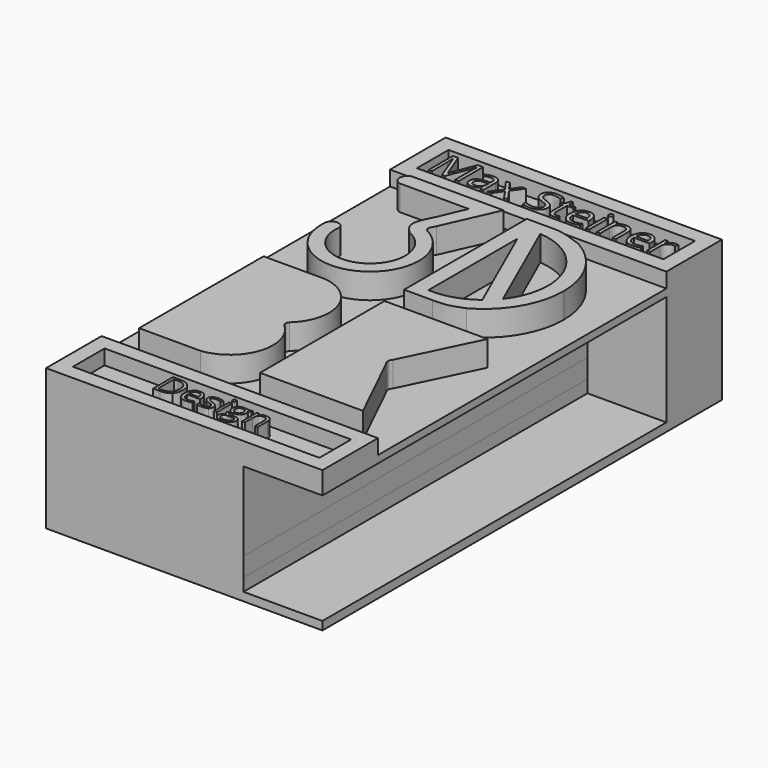
from build123d import *

# Parameters (mm, degrees)
F1_W         = 55.6107703596
F1_H         = 92.8997322917
F2_DEPTH     = 25.4
F3_DEPTH     = 5.08
F4_TEXT_SIZE = 8.577041121
F5_DEPTH     = 3
F4_W         = 0.5673257474
F4_H         = 3.7439126875
F6_DEPTH     = 3
F7_W         = 55.6107703596
F7_H         = 3.7946861994
F8_DEPTH     = 25.4
F9_W         = 55.6107703596
F9_H         = 3.7949544203
F10_DEPTH    = 25.4
F11_W        = 15.875
F11_H        = 7.9375
F11_W_2      = 15.8749995753
F11_H_2      = 3.81
F12_DEPTH    = 86.5193729115


# Not quite as in the source:
# - ends of sketch curves that miss each other by under 0.0002 mm in the source are joined
# - Text() gives the source's letters only with a copy of the font that has no kerning and outlines rounded to 1/6400 em; it was checked with that copy


with BuildPart() as f2:
    # F1 (on Top) → F2 (new body)
    with BuildSketch(Plane.XY):
        with Locations((-0.0001015142, 0.0001341105)):
            Rectangle(F1_W, F1_H)
    extrude(amount=-F2_DEPTH)

    # F0 (on Top) → F3 (join)
    with BuildSketch(Plane.XY):
        with BuildLine():
            Line((1.9535701722, 33.4806852043), (1.9535701722, 2.6171170175))
            Line((1.9535701722, 2.6171170175), (7.6673883013, 2.6171170175))
            add(Edge.make_bspline(
                [(13.5640528841, 3.8033656441), (12.5585792201, 3.4051600509), (10.5947152477, 2.6273956539), (8.6274422547, 2.6204880265), (7.6673883013, 2.6171170175)],
                knots=[0, 0, 0, 0, 0.5119874279, 1, 1, 1, 1], degree=3))
            ThreePointArc((13.5640528841, 3.8033656441), (19.5771167094, 9.6257290209), (21.8482203782, 17.6817168551))
            Line((21.8482203782, 17.6817168551), (21.8482203782, 18.0489011109))
            ThreePointArc((21.8482203782, 18.0489011109), (19.5771167094, 26.1048889451), (13.5640528841, 31.9272523219))
            add(Edge.make_bspline(
                [(13.5640528841, 31.9272523219), (12.0188625137, 32.4806988664), (9.5071250594, 33.3803371514), (8.1786150797, 33.4528004476), (7.6673883013, 33.4806852043)],
                knots=[0, 0, 0, 0, 0.6151878524, 1, 1, 1, 1], degree=3))
            Line((7.6673883013, 33.4806852043), (1.9535701722, 33.4806852043))
        make_face()
        with BuildLine():
            ThreePointArc((13.7255926495, 7.5781230036), (9.6198125415, 5.4448354943), (5.0269701927, 4.8843490524))
            Line((5.0269701927, 4.8843490524), (5.0269701927, 27.2558980547))
            Line((5.0269701927, 27.2558980547), (13.7255926495, 7.5781230036))
        make_face(mode=Mode.SUBTRACT)
        with BuildLine():
            ThreePointArc((6.7811124511, 30.8286115181), (17.6657420253, 23.1223286699), (16.0391214303, 9.8854082672))
            Line((16.0391214303, 9.8854082672), (6.7811124511, 30.8286115181))
        make_face(mode=Mode.SUBTRACT)
        with BuildLine():
            Line((-7.5453622267, 22.6989928633), (-2.7351737954, 33.4806852043))
            Line((-2.7351737954, 33.4806852043), (-21.1572051048, 33.4806852043))
            ThreePointArc((-21.1572051048, 33.4806852043), (-22.3890896886, 31.9530339911), (-21.1572051048, 30.425382778))
            Line((-21.1572051048, 30.425382778), (-7.2931135073, 30.425382778))
            Line((-7.2931135073, 30.425382778), (-9.4495294616, 25.3879800439))
            add(Edge.make_bspline(
                [(-9.4495294616, 25.3879800439), (-10.3302159731, 23.6726618568), (-11.8808970013, 20.6523914937), (-10.1830913379, 19.0052173822), (-9.4495294616, 18.2935316116)],
                knots=[0, 0, 0, 0, 0.5679353107, 1, 1, 1, 1], degree=3))
            ThreePointArc((-9.4495294616, 18.2935316116), (-8.744805336, 5.5966861339), (-19.1914085299, 12.8475483507))
            ThreePointArc((-19.1914085299, 12.8475483507), (-20.5873309935, 13.9352987723), (-21.9832534571, 12.8475483507))
            ThreePointArc((-21.9832534571, 12.8475483507), (-7.5716745464, 3.0830422585), (-7.6246123494, 20.4909825018))
            add(Edge.make_bspline(
                [(-7.5453622267, 22.6989928633), (-7.8757345138, 22.1285959519), (-8.4306078493, 21.1705917574), (-7.8693930702, 20.681447967), (-7.6246123494, 20.4909825018)],
                knots=[0, 0, 0, 0, 0.5706142153, 0.9583691649, 0.9583691649, 0.9583691649, 0.9583691649], degree=3))
        make_face()
        with BuildLine():
            Line((1.9535701722, -33.6182080209), (21.8482203782, -33.6182080209))
            Line((21.8482203782, -33.6182080209), (22.670282051, -33.6182080209))
            Line((22.670282051, -33.6182080209), (15.4876355082, -18.8196848612))
            add(Edge.make_bspline(
                [(15.4876355082, -18.8196848612), (15.371168109, -18.6560732739), (15.159509665, -18.3587387901), (15.1679139181, -18.0863425739), (15.171693638, -17.9638353875)],
                knots=[0, 0, 0, 0, 0.550261057, 1, 1, 1, 1], degree=3))
            add(Edge.make_bspline(
                [(15.4876355082, -17.1079859138), (15.371168109, -17.2715975011), (15.159509665, -17.5689319849), (15.1679139181, -17.8413282011), (15.171693638, -17.9638353875)],
                knots=[0, 0, 0, 0, 0.550261057, 1, 1, 1, 1], degree=3))
            Line((15.4876355082, -17.1079859138), (22.670282051, -2.3094627541))
            Line((22.670282051, -2.3094627541), (1.9535701722, -2.3094627541))
            Line((1.9535701722, -2.3094627541), (1.9535701722, -33.6182080209))
        make_face()
        with BuildLine():
            Line((-22.3890896886, -2.3094627541), (-22.3890896886, -33.6182080209))
            Line((-22.3890896886, -33.6182080209), (-10.0687015802, -33.6182080209))
            ThreePointArc((-10.0687015802, -33.6182080209), (-2.7489802993, -27.706179837), (-5.1699676551, -18.6139184516))
            add(Edge.make_bspline(
                [(-5.1699676551, -18.6139184516), (-5.2577137292, -18.4897791328), (-5.4173213156, -18.2639732804), (-5.4122223799, -18.0570156997), (-5.4099266417, -17.9638353875)],
                knots=[0, 0, 0, 0, 0.5497612996, 1, 1, 1, 1], degree=3))
            add(Edge.make_bspline(
                [(-5.1699676551, -17.3137523234), (-5.2577137292, -17.4378916422), (-5.4173213156, -17.6636974946), (-5.4122223799, -17.8706550753), (-5.4099266417, -17.9638353875)],
                knots=[0, 0, 0, 0, 0.5497612996, 1, 1, 1, 1], degree=3))
            ThreePointArc((-5.1699676551, -17.3137523234), (-2.7489802993, -8.221490938), (-10.0687015802, -2.3094627541))
            Line((-10.0687015802, -2.3094627541), (-22.3890896886, -2.3094627541))
        make_face()
    extrude(amount=F3_DEPTH)

    # F4 (on face) → F5 (join)
    with BuildSketch(Plane.XY):
        with Locations((-23.8402802497, 39.9415232241)):
            Text('Max Steiner', F4_TEXT_SIZE, font='Open Sans', text_align=(TextAlign.LEFT, TextAlign.BOTTOM))
        Polygon((-27.805486694, 46.4500002563), (-27.805486694, 36.2746864557), (27.8052836657, 36.2746864557), (27.8052836657, 46.4500002563), (24.8052836657, 46.4500002563), (24.8052836657, 39.2746864557), (-24.805486694, 39.2746864557), (-24.805486694, 46.4500002563), align=None)
        Polygon((-27.805486694, 50.2446864557), (-27.805486694, 46.4500002563), (-24.805486694, 46.4500002563), (-24.805486694, 47.2446864557), (24.8052836657, 47.2446864557), (24.8052836657, 46.4500002563), (27.8052836657, 46.4500002563), (27.8052836657, 50.2446864557), align=None)
    extrude(amount=F5_DEPTH)

    # F4 (on face) → F6 (join)
    with BuildSketch(Plane.XY):
        Polygon((27.8052836657, -36.2746864557), (-27.805486694, -36.2746864557), (-27.805486694, -46.4497320354), (-24.805486694, -46.4497320354), (-24.805486694, -39.2746864557), (24.8052836657, -39.2746864557), (24.8052836657, -46.4497320354), (27.8052836657, -46.4497320354), align=None)
        Polygon((-24.805486694, -46.4497320354), (-27.805486694, -46.4497320354), (-27.805486694, -50.2446864557), (27.8052836657, -50.2446864557), (27.8052836657, -46.4497320354), (24.8052836657, -46.4497320354), (24.8052836657, -47.2446864557), (-24.805486694, -47.2446864557), align=None)
        with BuildLine():
            add(Edge.make_bspline(
                [(-6.3295820825, -42.6227643038), (-6.3295820825, -43.8590753256), (-7.0007535833, -44.5133035719)],
                knots=[0, 0, 0, 1, 1, 1], degree=2))
            add(Edge.make_bspline(
                [(-6.9750654232, -40.818580978), (-6.3295820825, -41.4640643188), (-6.3295820825, -42.6227643038)],
                knots=[0, 0, 0, 1, 1, 1], degree=2))
            add(Edge.make_bspline(
                [(-8.7858074282, -40.1730976373), (-7.620548764, -40.1730976373), (-6.9750654232, -40.818580978)],
                knots=[0, 0, 0, 1, 1, 1], degree=2))
            Line((-8.7858074282, -40.1730976373), (-10.316165899, -40.1730976373))
            Line((-10.316165899, -40.1730976373), (-10.316165899, -45.1675318182))
            Line((-10.316165899, -45.1675318182), (-8.9322845961, -45.1675318182))
            add(Edge.make_bspline(
                [(-7.0007535833, -44.5133035719), (-7.671925084, -45.1675318182), (-8.9322845961, -45.1675318182)],
                knots=[0, 0, 0, 1, 1, 1], degree=2))
        make_face()
        with BuildLine():
            add(Edge.make_bspline(
                [(-6.9439116972, -42.6435334545), (-6.9439116972, -41.6662902596), (-7.4341729645, -41.1711099829)],
                knots=[0, 0, 0, 1, 1, 1], degree=2))
            add(Edge.make_bspline(
                [(-7.4669663603, -44.1547624444), (-6.9439116972, -43.6437320265), (-6.9439116972, -42.6435334545)],
                knots=[0, 0, 0, 1, 1, 1], degree=2))
            add(Edge.make_bspline(
                [(-9.0284785571, -44.6657928624), (-7.9900210233, -44.6657928624), (-7.4669663603, -44.1547624444)],
                knots=[0, 0, 0, 1, 1, 1], degree=2))
            Line((-9.0284785571, -44.6657928624), (-9.7357227933, -44.6657928624))
            Line((-9.7357227933, -44.6657928624), (-9.7357227933, -40.6759297063))
            Line((-9.7357227933, -40.6759297063), (-8.8918394079, -40.6759297063))
            add(Edge.make_bspline(
                [(-7.4341729645, -41.1711099829), (-7.9244342317, -40.6759297063), (-8.8918394079, -40.6759297063)],
                knots=[0, 0, 0, 1, 1, 1], degree=2))
        make_face(mode=Mode.SUBTRACT)
        with BuildLine():
            add(Edge.make_bspline(
                [(-3.7192277766, -45.2363979493), (-4.5489006904, -45.2363979493), (-5.0293239389, -44.7302865408)],
                knots=[0, 0, 0, 1, 1, 1], degree=2))
            add(Edge.make_bspline(
                [(-3.072104766, -45.1795560633), (-3.3399174984, -45.2363979493), (-3.7192277766, -45.2363979493)],
                knots=[0, 0, 0, 1, 1, 1], degree=2))
            add(Edge.make_bspline(
                [(-2.5036859054, -44.9937268204), (-2.8042920336, -45.1227141772), (-3.072104766, -45.1795560633)],
                knots=[0, 0, 0, 1, 1, 1], degree=2))
            Line((-2.5036859054, -44.9937268204), (-2.5036859054, -44.4876154118))
            add(Edge.make_bspline(
                [(-3.6984586259, -44.7401245595), (-3.0939670299, -44.7401245595), (-2.5036859054, -44.4876154118)],
                knots=[0, 0, 0, 1, 1, 1], degree=2))
            add(Edge.make_bspline(
                [(-4.5882527653, -44.3985266866), (-4.2723430524, -44.7401245595), (-3.6984586259, -44.7401245595)],
                knots=[0, 0, 0, 1, 1, 1], degree=2))
            add(Edge.make_bspline(
                [(-4.9216522893, -43.397781558), (-4.9041624782, -44.0569288136), (-4.5882527653, -44.3985266866)],
                knots=[0, 0, 0, 1, 1, 1], degree=2))
            Line((-4.9216522893, -43.397781558), (-2.342998266, -43.397781558))
            Line((-2.342998266, -43.397781558), (-2.342998266, -43.0392404305))
            add(Edge.make_bspline(
                [(-2.7529157135, -41.8176864368), (-2.342998266, -42.2806198743), (-2.342998266, -43.0392404305)],
                knots=[0, 0, 0, 1, 1, 1], degree=2))
            add(Edge.make_bspline(
                [(-3.8657049445, -41.3547529994), (-3.1628331611, -41.3547529994), (-2.7529157135, -41.8176864368)],
                knots=[0, 0, 0, 1, 1, 1], degree=2))
            add(Edge.make_bspline(
                [(-5.0637570045, -41.8876456812), (-4.6177668216, -41.3547529994), (-3.8657049445, -41.3547529994)],
                knots=[0, 0, 0, 1, 1, 1], degree=2))
            add(Edge.make_bspline(
                [(-5.5097471874, -43.3267292004), (-5.5097471874, -42.420538363), (-5.0637570045, -41.8876456812)],
                knots=[0, 0, 0, 1, 1, 1], degree=2))
            add(Edge.make_bspline(
                [(-5.0293239389, -44.7302865408), (-5.5097471874, -44.2241751322), (-5.5097471874, -43.3267292004)],
                knots=[0, 0, 0, 1, 1, 1], degree=2))
        make_face()
        with BuildLine():
            add(Edge.make_bspline(
                [(-3.8733567368, -41.8302572386), (-4.3237193725, -41.8302572386), (-4.5920786615, -42.123758131)],
                knots=[0, 0, 0, 1, 1, 1], degree=2))
            add(Edge.make_bspline(
                [(-3.1896144343, -42.1155597821), (-3.4284596671, -41.8302572386), (-3.8733567368, -41.8302572386)],
                knots=[0, 0, 0, 1, 1, 1], degree=2))
            add(Edge.make_bspline(
                [(-2.9507692016, -42.9364877903), (-2.9507692016, -42.4008623255), (-3.1896144343, -42.1155597821)],
                knots=[0, 0, 0, 1, 1, 1], degree=2))
            Line((-2.9507692016, -42.9364877903), (-4.908534931, -42.9364877903))
            add(Edge.make_bspline(
                [(-4.5920786615, -42.123758131), (-4.8604379505, -42.4172590234), (-4.908534931, -42.9364877903)],
                knots=[0, 0, 0, 1, 1, 1], degree=2))
        make_face(mode=Mode.SUBTRACT)
        with BuildLine():
            add(Edge.make_bspline(
                [(1.0390939545, -44.1465640955), (1.0390939545, -44.6690722019), (0.6499456576, -44.9527350756)],
                knots=[0, 0, 0, 1, 1, 1], degree=2))
            add(Edge.make_bspline(
                [(0.8051677311, -43.527862028), (1.0390939545, -43.7738124965), (1.0390939545, -44.1465640955)],
                knots=[0, 0, 0, 1, 1, 1], degree=2))
            add(Edge.make_bspline(
                [(-0.0944644271, -43.0392404305), (0.5712415077, -43.2819115595), (0.8051677311, -43.527862028)],
                knots=[0, 0, 0, 1, 1, 1], degree=2))
            add(Edge.make_bspline(
                [(-0.7503323432, -42.762136236), (-0.579806685, -42.8577836404), (-0.0944644271, -43.0392404305)],
                knots=[0, 0, 0, 1, 1, 1], degree=2))
            add(Edge.make_bspline(
                [(-0.9979224815, -42.5610034084), (-0.9208580013, -42.6664888316), (-0.7503323432, -42.762136236)],
                knots=[0, 0, 0, 1, 1, 1], degree=2))
            add(Edge.make_bspline(
                [(-1.0749869616, -42.3046683645), (-1.0749869616, -42.4555179852), (-0.9979224815, -42.5610034084)],
                knots=[0, 0, 0, 1, 1, 1], degree=2))
            add(Edge.make_bspline(
                [(-0.8700282378, -41.9565118124), (-1.0749869616, -42.0827663863), (-1.0749869616, -42.3046683645)],
                knots=[0, 0, 0, 1, 1, 1], degree=2))
            add(Edge.make_bspline(
                [(-0.2617107457, -41.8302572386), (-0.6650695141, -41.8302572386), (-0.8700282378, -41.9565118124)],
                knots=[0, 0, 0, 1, 1, 1], degree=2))
            add(Edge.make_bspline(
                [(0.759256977, -42.0619972356), (0.1963036824, -41.8302572386), (-0.2617107457, -41.8302572386)],
                knots=[0, 0, 0, 1, 1, 1], degree=2))
            Line((0.759256977, -42.0619972356), (0.9614829178, -41.6007034679))
            add(Edge.make_bspline(
                [(-0.2212655575, -41.3547529994), (0.3832260384, -41.3547529994), (0.9614829178, -41.6007034679)],
                knots=[0, 0, 0, 1, 1, 1], degree=2))
            add(Edge.make_bspline(
                [(-1.2422332802, -41.6198329488), (-0.8694816812, -41.3547529994), (-0.2212655575, -41.3547529994)],
                knots=[0, 0, 0, 1, 1, 1], degree=2))
            add(Edge.make_bspline(
                [(-1.6149848792, -42.3429273263), (-1.6149848792, -41.8849128982), (-1.2422332802, -41.6198329488)],
                knots=[0, 0, 0, 1, 1, 1], degree=2))
            add(Edge.make_bspline(
                [(-1.5073132296, -42.7829053867), (-1.6149848792, -42.5987158136), (-1.6149848792, -42.3429273263)],
                knots=[0, 0, 0, 1, 1, 1], degree=2))
            add(Edge.make_bspline(
                [(-1.1793792716, -43.1124790145), (-1.3996415801, -42.9670949597), (-1.5073132296, -42.7829053867)],
                knots=[0, 0, 0, 1, 1, 1], degree=2))
            add(Edge.make_bspline(
                [(-0.4366088566, -43.4524372176), (-0.9591169631, -43.2578630692), (-1.1793792716, -43.1124790145)],
                knots=[0, 0, 0, 1, 1, 1], degree=2))
            add(Edge.make_bspline(
                [(0.3034287753, -43.8197232506), (0.1143201929, -43.6645011772), (-0.4366088566, -43.4524372176)],
                knots=[0, 0, 0, 1, 1, 1], degree=2))
            add(Edge.make_bspline(
                [(0.4925373578, -44.1935679628), (0.4925373578, -43.9749453241), (0.3034287753, -43.8197232506)],
                knots=[0, 0, 0, 1, 1, 1], degree=2))
            add(Edge.make_bspline(
                [(0.253692125, -44.6258942308), (0.4925373578, -44.4843360722), (0.4925373578, -44.1935679628)],
                knots=[0, 0, 0, 1, 1, 1], degree=2))
            add(Edge.make_bspline(
                [(-0.4289570643, -44.7674523894), (0.0148468923, -44.7674523894), (0.253692125, -44.6258942308)],
                knots=[0, 0, 0, 1, 1, 1], degree=2))
            add(Edge.make_bspline(
                [(-1.0252503113, -44.689294796), (-0.7164458342, -44.7674523894), (-0.4289570643, -44.7674523894)],
                knots=[0, 0, 0, 1, 1, 1], degree=2))
            add(Edge.make_bspline(
                [(-1.6040537472, -44.4744980535), (-1.3340547885, -44.6111372027), (-1.0252503113, -44.689294796)],
                knots=[0, 0, 0, 1, 1, 1], degree=2))
            Line((-1.6040537472, -44.4744980535), (-1.6040537472, -45.0002854996))
            add(Edge.make_bspline(
                [(-0.4431675358, -45.2363979493), (-1.1875776205, -45.2363979493), (-1.6040537472, -45.0002854996)],
                knots=[0, 0, 0, 1, 1, 1], degree=2))
            add(Edge.make_bspline(
                [(0.6499456576, -44.9527350756), (0.2607973608, -45.2363979493), (-0.4431675358, -45.2363979493)],
                knots=[0, 0, 0, 1, 1, 1], degree=2))
        make_face()
        with Locations((2.2453443635, -43.2955754744)):
            Rectangle(F4_W, F4_H)
        with BuildLine():
            add(Edge.make_bspline(
                [(1.9135845093, -40.4092100871), (1.9135845093, -40.2146359387), (2.0092319137, -40.1239075436)],
                knots=[0, 0, 0, 1, 1, 1], degree=2))
            add(Edge.make_bspline(
                [(2.0092319137, -40.6945126306), (1.9135845093, -40.6005048959), (1.9135845093, -40.4092100871)],
                knots=[0, 0, 0, 1, 1, 1], degree=2))
            add(Edge.make_bspline(
                [(2.2491702597, -40.7885203652), (2.1048793181, -40.7885203652), (2.0092319137, -40.6945126306)],
                knots=[0, 0, 0, 1, 1, 1], degree=2))
            add(Edge.make_bspline(
                [(2.4847361528, -40.6945126306), (2.3858094088, -40.7885203652), (2.2491702597, -40.7885203652)],
                knots=[0, 0, 0, 1, 1, 1], degree=2))
            add(Edge.make_bspline(
                [(2.5836628968, -40.4092100871), (2.5836628968, -40.6005048959), (2.4847361528, -40.6945126306)],
                knots=[0, 0, 0, 1, 1, 1], degree=2))
            add(Edge.make_bspline(
                [(2.4847361528, -40.1255472134), (2.5836628968, -40.2179152782), (2.5836628968, -40.4092100871)],
                knots=[0, 0, 0, 1, 1, 1], degree=2))
            add(Edge.make_bspline(
                [(2.2491702597, -40.0331791485), (2.3858094088, -40.0331791485), (2.4847361528, -40.1255472134)],
                knots=[0, 0, 0, 1, 1, 1], degree=2))
            add(Edge.make_bspline(
                [(2.0092319137, -40.1239075436), (2.1048793181, -40.0331791485), (2.2491702597, -40.0331791485)],
                knots=[0, 0, 0, 1, 1, 1], degree=2))
        make_face()
        with BuildLine():
            Line((10.1261439316, -42.7451929815), (10.1261439316, -45.1675318182))
            Line((10.1261439316, -45.1675318182), (10.693469679, -45.1675318182))
            Line((10.693469679, -45.1675318182), (10.693469679, -42.725516944))
            add(Edge.make_bspline(
                [(10.3518718061, -41.6810472877), (10.693469679, -42.0073415759), (10.693469679, -42.725516944)],
                knots=[0, 0, 0, 1, 1, 1], degree=2))
            add(Edge.make_bspline(
                [(9.3336368664, -41.3547529994), (10.0102739331, -41.3547529994), (10.3518718061, -41.6810472877)],
                knots=[0, 0, 0, 1, 1, 1], degree=2))
            add(Edge.make_bspline(
                [(8.633497866, -41.5072422899), (8.9477679091, -41.3547529994), (9.3336368664, -41.3547529994)],
                knots=[0, 0, 0, 1, 1, 1], degree=2))
            add(Edge.make_bspline(
                [(8.1443297119, -41.9362892183), (8.3192278228, -41.6597315804), (8.633497866, -41.5072422899)],
                knots=[0, 0, 0, 1, 1, 1], degree=2))
            Line((8.1443297119, -41.9362892183), (8.1170018821, -41.9362892183))
            Line((8.1170018821, -41.9362892183), (8.0251803738, -41.4236191306))
            Line((8.0251803738, -41.4236191306), (7.5638866062, -41.4236191306))
            Line((7.5638866062, -41.4236191306), (7.5638866062, -45.1675318182))
            Line((7.5638866062, -45.1675318182), (8.1312123536, -45.1675318182))
            Line((8.1312123536, -45.1675318182), (8.1312123536, -43.2032074095))
            add(Edge.make_bspline(
                [(8.4044906519, -42.1543653004), (8.1312123536, -42.4719146831), (8.1312123536, -43.2032074095)],
                knots=[0, 0, 0, 1, 1, 1], degree=2))
            add(Edge.make_bspline(
                [(9.2647707352, -41.8368159177), (8.6777689503, -41.8368159177), (8.4044906519, -42.1543653004)],
                knots=[0, 0, 0, 1, 1, 1], degree=2))
            add(Edge.make_bspline(
                [(9.9179058683, -42.0625437922), (9.7096678049, -41.8368159177), (9.2647707352, -41.8368159177)],
                knots=[0, 0, 0, 1, 1, 1], degree=2))
            add(Edge.make_bspline(
                [(10.1261439316, -42.7451929815), (10.1261439316, -42.2882716666), (9.9179058683, -42.0625437922)],
                knots=[0, 0, 0, 1, 1, 1], degree=2))
        make_face()
        with BuildLine():
            add(Edge.make_bspline(
                [(3.5109515035, -46.4497320354), (3.2635793032, -46.196519284), (3.2635793032, -45.8026305835)],
                knots=[0.2115172688, 0.2115172688, 0.2115172688, 1, 1, 1], degree=2))
            Line((3.5109515035, -46.4497320354), (6.3492143086, -46.4497320354))
            add(Edge.make_bspline(
                [(6.7473310507, -45.5741699261), (6.7473310507, -46.1300327557), (6.3492143086, -46.4497320354)],
                knots=[0, 0, 0, 0.8936968585, 0.8936968585, 0.8936968585], degree=2))
            add(Edge.make_bspline(
                [(6.421583319, -44.8292132848), (6.7473310507, -45.0855483286), (6.7473310507, -45.5741699261)],
                knots=[0, 0, 0, 1, 1, 1], degree=2))
            add(Edge.make_bspline(
                [(5.4869715386, -44.5728782409), (6.0958355874, -44.5728782409), (6.421583319, -44.8292132848)],
                knots=[0, 0, 0, 1, 1, 1], degree=2))
            Line((5.4869715386, -44.5728782409), (4.8245449434, -44.5728782409))
            add(Edge.make_bspline(
                [(4.3911255622, -44.499639657), (4.517380136, -44.5728782409), (4.8245449434, -44.5728782409)],
                knots=[0, 0, 0, 1, 1, 1], degree=2))
            add(Edge.make_bspline(
                [(4.2648709884, -44.2722721127), (4.2648709884, -44.426401073), (4.3911255622, -44.499639657)],
                knots=[0, 0, 0, 1, 1, 1], degree=2))
            add(Edge.make_bspline(
                [(4.6266914554, -43.7913023076), (4.2648709884, -43.9825971165), (4.2648709884, -44.2722721127)],
                knots=[0, 0, 0, 1, 1, 1], degree=2))
            add(Edge.make_bspline(
                [(4.9404149419, -43.8186301374), (4.7731686233, -43.8186301374), (4.6266914554, -43.7913023076)],
                knots=[0, 0, 0, 1, 1, 1], degree=2))
            add(Edge.make_bspline(
                [(5.9723137965, -43.4906961794), (5.596282858, -43.8186301374), (4.9404149419, -43.8186301374)],
                knots=[0, 0, 0, 1, 1, 1], degree=2))
            add(Edge.make_bspline(
                [(6.3483447351, -42.6118331719), (6.3483447351, -43.1627622214), (5.9723137965, -43.4906961794)],
                knots=[0, 0, 0, 1, 1, 1], degree=2))
            add(Edge.make_bspline(
                [(6.2729199247, -42.1767741209), (6.3483447351, -42.3702551561), (6.3483447351, -42.6118331719)],
                knots=[0, 0, 0, 1, 1, 1], degree=2))
            add(Edge.make_bspline(
                [(6.1023942665, -41.8641437476), (6.1974951144, -41.9832930857), (6.2729199247, -42.1767741209)],
                knots=[0, 0, 0, 1, 1, 1], degree=2))
            Line((6.1023942665, -41.8641437476), (6.7954280312, -41.7821602581))
            Line((6.7954280312, -41.7821602581), (6.7954280312, -41.4236191306))
            Line((6.7954280312, -41.4236191306), (5.5011820101, -41.4236191306))
            add(Edge.make_bspline(
                [(4.9710221113, -41.3547529994), (5.2650695604, -41.3547529994), (5.5011820101, -41.4236191306)],
                knots=[0, 0, 0, 1, 1, 1], degree=2))
            add(Edge.make_bspline(
                [(3.926552455, -41.6881525234), (4.2954781578, -41.3547529994), (4.9710221113, -41.3547529994)],
                knots=[0, 0, 0, 1, 1, 1], degree=2))
            add(Edge.make_bspline(
                [(3.5576267522, -42.6358816621), (3.5576267522, -42.0215520474), (3.926552455, -41.6881525234)],
                knots=[0, 0, 0, 1, 1, 1], degree=2))
            add(Edge.make_bspline(
                [(3.7401766555, -43.2922961348), (3.5576267522, -43.0053539215), (3.5576267522, -42.6358816621)],
                knots=[0, 0, 0, 1, 1, 1], degree=2))
            add(Edge.make_bspline(
                [(4.2134946683, -43.6983876862), (3.9227265588, -43.5792383481), (3.7401766555, -43.2922961348)],
                knots=[0, 0, 0, 1, 1, 1], degree=2))
            add(Edge.make_bspline(
                [(3.8680708991, -43.9957144748), (3.9773822185, -43.8415855145), (4.2134946683, -43.6983876862)],
                knots=[0, 0, 0, 1, 1, 1], degree=2))
            add(Edge.make_bspline(
                [(3.7587595798, -44.3542556022), (3.7587595798, -44.1498434351), (3.8680708991, -43.9957144748)],
                knots=[0, 0, 0, 1, 1, 1], degree=2))
            add(Edge.make_bspline(
                [(3.856046654, -44.6723515415), (3.7587595798, -44.5357123923), (3.7587595798, -44.3542556022)],
                knots=[0, 0, 0, 1, 1, 1], degree=2))
            add(Edge.make_bspline(
                [(4.0965315566, -44.8734843691), (3.9533337282, -44.8089906907), (3.856046654, -44.6723515415)],
                knots=[0, 0, 0, 1, 1, 1], degree=2))
            add(Edge.make_bspline(
                [(3.4822019419, -45.2118029025), (3.7008245805, -44.9620265378), (4.0965315566, -44.8734843691)],
                knots=[0, 0, 0, 1, 1, 1], degree=2))
            add(Edge.make_bspline(
                [(3.2635793032, -45.8026305835), (3.2635793032, -45.4615792672), (3.4822019419, -45.2118029025)],
                knots=[0, 0, 0, 1, 1, 1], degree=2))
        make_face()
        with BuildLine():
            add(Edge.make_bspline(
                [(3.8101358999, -45.7960719044), (3.8101358999, -46.0999573722), (4.0664709438, -46.257365672)],
                knots=[0, 0, 0, 1, 1, 1], degree=2))
            add(Edge.make_bspline(
                [(4.025479199, -45.2664585622), (3.8101358999, -45.4506481353), (3.8101358999, -45.7960719044)],
                knots=[0, 0, 0, 1, 1, 1], degree=2))
            add(Edge.make_bspline(
                [(4.6266914554, -45.0822689891), (4.2408224981, -45.0822689891), (4.025479199, -45.2664585622)],
                knots=[0, 0, 0, 1, 1, 1], degree=2))
            Line((4.6266914554, -45.0822689891), (5.3066078617, -45.0822689891))
            add(Edge.make_bspline(
                [(6.0133055413, -45.200325214), (5.8258366286, -45.0822689891), (5.3066078617, -45.0822689891)],
                knots=[0, 0, 0, 1, 1, 1], degree=2))
            add(Edge.make_bspline(
                [(6.2007744539, -45.6222669066), (6.2007744539, -45.3183814388), (6.0133055413, -45.200325214)],
                knots=[0, 0, 0, 1, 1, 1], degree=2))
            add(Edge.make_bspline(
                [(5.8575369112, -46.2010703426), (6.2007744539, -45.9873667132), (6.2007744539, -45.6222669066)],
                knots=[0, 0, 0, 1, 1, 1], degree=2))
            add(Edge.make_bspline(
                [(4.8004964531, -46.4147739719), (5.5142993685, -46.4147739719), (5.8575369112, -46.2010703426)],
                knots=[0, 0, 0, 1, 1, 1], degree=2))
            add(Edge.make_bspline(
                [(4.0664709438, -46.257365672), (4.3228059876, -46.4147739719), (4.8004964531, -46.4147739719)],
                knots=[0, 0, 0, 1, 1, 1], degree=2))
        make_face(mode=Mode.SUBTRACT)
        with BuildLine():
            add(Edge.make_bspline(
                [(4.1173007072, -42.6227643038), (4.1173007072, -43.0151919403), (4.3392026855, -43.2168713245)],
                knots=[0, 0, 0, 1, 1, 1], degree=2))
            add(Edge.make_bspline(
                [(4.3326440064, -41.9838396422), (4.1173007072, -42.1986363848), (4.1173007072, -42.6227643038)],
                knots=[0, 0, 0, 1, 1, 1], degree=2))
            add(Edge.make_bspline(
                [(4.9480667343, -41.7690428997), (4.5479873055, -41.7690428997), (4.3326440064, -41.9838396422)],
                knots=[0, 0, 0, 1, 1, 1], degree=2))
            add(Edge.make_bspline(
                [(5.7875776668, -42.6118331719), (5.7875776668, -41.7690428997), (4.9480667343, -41.7690428997)],
                knots=[0, 0, 0, 1, 1, 1], degree=2))
            add(Edge.make_bspline(
                [(4.957904753, -43.4185507086), (5.7875776668, -43.4185507086), (5.7875776668, -42.6118331719)],
                knots=[0, 0, 0, 1, 1, 1], degree=2))
            add(Edge.make_bspline(
                [(4.3392026855, -43.2168713245), (4.5611046638, -43.4185507086), (4.957904753, -43.4185507086)],
                knots=[0, 0, 0, 1, 1, 1], degree=2))
        make_face(mode=Mode.SUBTRACT)
        with BuildLine():
            Line((6.3492143086, -46.4497320354), (3.5109515035, -46.4497320354))
            add(Edge.make_bspline(
                [(3.6614725056, -46.5754616113), (3.5773112221, -46.517658532), (3.5109515035, -46.4497320354)],
                knots=[0, 0, 0, 0.2115172688, 0.2115172688, 0.2115172688], degree=2))
            add(Edge.make_bspline(
                [(4.793937774, -46.8487399097), (4.059365708, -46.8487399097), (3.6614725056, -46.5754616113)],
                knots=[0, 0, 0, 1, 1, 1], degree=2))
            add(Edge.make_bspline(
                [(6.2488714345, -46.5224456214), (5.7504118183, -46.8487399097), (4.793937774, -46.8487399097)],
                knots=[0, 0, 0, 1, 1, 1], degree=2))
            add(Edge.make_bspline(
                [(6.3492143086, -46.4497320354), (6.3018592576, -46.4877595135), (6.2488714345, -46.5224456214)],
                knots=[0.8936968585, 0.8936968585, 0.8936968585, 1, 1, 1], degree=2))
        make_face()
    extrude(amount=F6_DEPTH)

    # F7 (on face) → F8 (join, through all)
    with BuildSketch(Plane(origin=(0, 0, 0), x_dir=(1, 0, 0), z_dir=(0, 0, -1))):
        with Locations((-0.0001015142, -48.347343356)):
            Rectangle(F7_W, F7_H)
    extrude(amount=F8_DEPTH)

    # F9 (on face) → F10 (join, through all)
    with BuildSketch(Plane(origin=(0, 0, 0), x_dir=(1, 0, 0), z_dir=(0, 0, -1))):
        with Locations((-0.0001015142, 48.3472092456)):
            Rectangle(F9_W, F9_H)
    extrude(amount=F10_DEPTH)

    # F11 (on face) → F12 (cut, through all)
    with BuildSketch(Plane.XZ.offset(50.2446864557)):
        with Locations((19.8677840903, -5.4532486349)):
            Rectangle(F11_W, F11_H)
        with Locations((19.867783878, -13.3907486349)):
            Rectangle(F11_W_2, F11_H)
        with Locations((19.867783878, -19.2644986349)):
            Rectangle(F11_W_2, F11_H_2)
        Polygon((11.9302840903, -23.7094986349), (27.8052840903, -23.7094986349), (27.8052836657, -21.1694986349), (11.9302840903, -21.1694986349), (11.9302840903, -22.4394986349), align=None)
    extrude(amount=-F12_DEPTH, mode=Mode.SUBTRACT)


solid = f2.part
